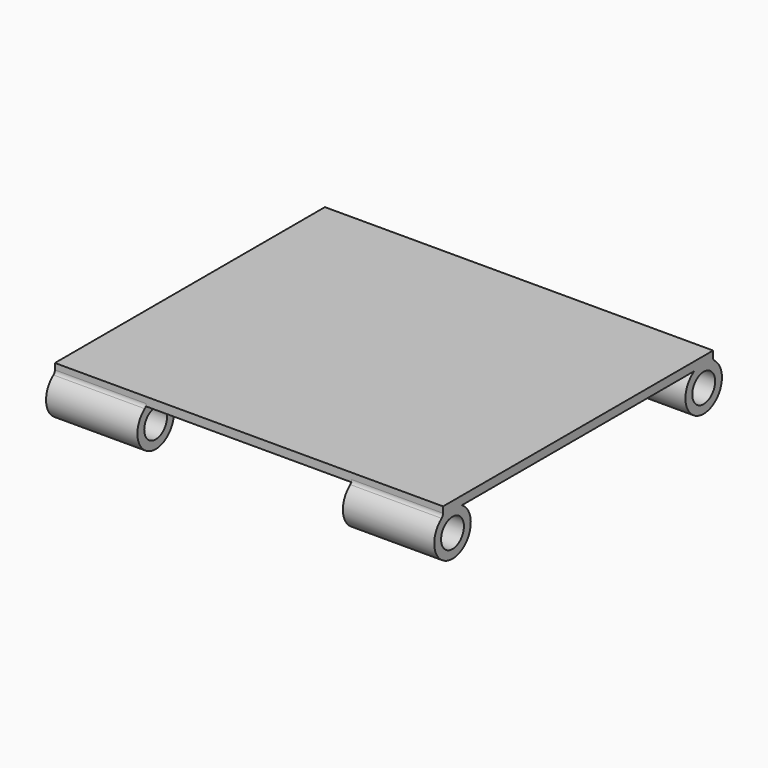
from build123d import *

# Parameters (mm, degrees)
F0_R          = 15.875
F1_DEPTH      = 431.8
F3_DEPTH      = 67.056
F3_DEPTH_BACK = 51.816
F6_R          = 5.08


# Not quite as in the source:
# - a feature of the source that left no trace in its solid (it failed there, or was rolled back) is left out


with BuildPart() as f1:
    # F0 (on Right) → F1 (new body)
    with BuildSketch(Plane.YZ):
        with BuildLine():
            Line((-342.5169996576, 21.7714285714), (-13.0830003424, 21.7714285714))
            ThreePointArc((-13.0830003424, 21.7714285714), (0, -25.4), (13.0830003424, 21.7714285714))
            Line((13.0830003424, 21.7714285714), (13.0830003424, 31.2964285714))
            Line((13.0830003424, 31.2964285714), (-342.5169996576, 31.2964285714))
            Line((-342.5169996576, 31.2964285714), (-342.5169996576, 24.9464285714))
            Line((-342.5169996576, 24.9464285714), (-342.5169996576, 21.7714285714))
        make_face()
        Circle(F0_R, mode=Mode.SUBTRACT)
    extrude(amount=F1_DEPTH)

    # F2 (on face) → F3 (cut, two sides)
    with BuildSketch(Plane(origin=(0, 13.0830003424, 0), x_dir=(-1, 0, 0), z_dir=(0, 1, 0))) as f3_sk:
        Polygon((-101.6, 21.7714285714), (-215.9, 21.7714285714), (-330.2, 21.7714285714), (-330.2, -30.4525513202), (-228.6, -30.4525513202), (-101.6, -30.4525513202), align=None)
    extrude(amount=-F3_DEPTH, mode=Mode.SUBTRACT)
    extrude(f3_sk.sketch, amount=F3_DEPTH_BACK, mode=Mode.SUBTRACT)

    # F5: F1 across plane


with BuildPart() as f1_1:
    add(f1.part)
    add(f1.part.mirror(Plane.XZ.offset(174.625)))

    # F6
    f6_edges = [f1_1.edges().sort_by_distance(p)[0] for p in [
        (50.8, -362.333, 21.771429),
        (381, -362.333, 21.771429),
        (50.8, 13.083, 21.771429),
        (381, 13.083, 21.771429),
    ]]
    fillet(f6_edges, radius=F6_R)


solid = f1_1.part
